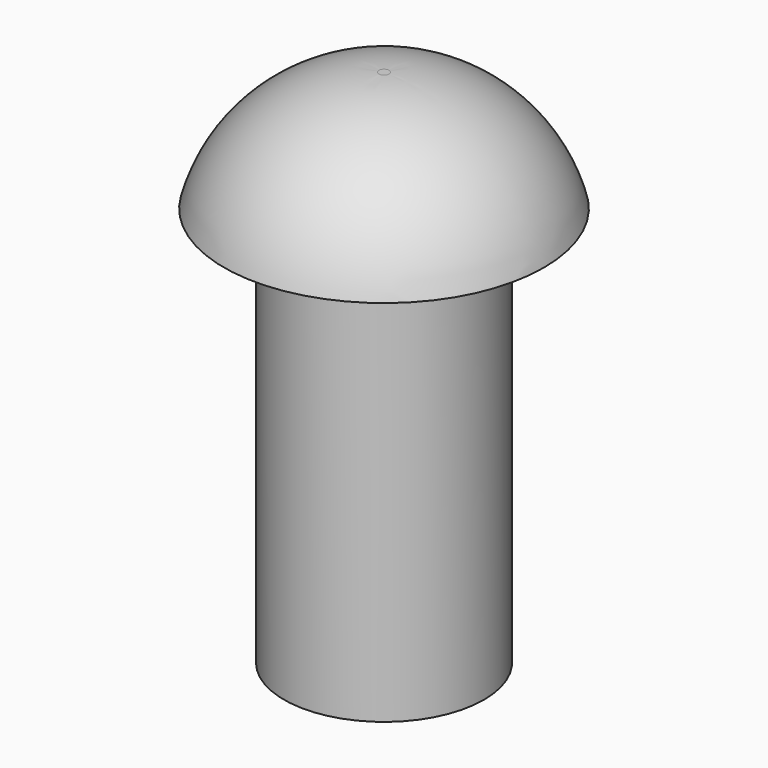
from build123d import *

# Parameters (mm, degrees)
F0_R     = 3.175
F1_DEPTH = 12.7
F2_R     = 5.08
F3_DEPTH = 3.81


# Not quite as in the source:
# - a fillet or chamfer that OpenCascade refuses, or shapes differently, is made with other operations: its cross-section is extruded or revolved along the edge and cut away or added


with BuildPart() as f1:
    # F0 (on Top) → F1 (new body)
    with BuildSketch(Plane.XY):
        with Locations((-67.7428916097, -29.48333323)):
            Circle(F0_R)
    extrude(amount=F1_DEPTH)

    # F2 (on face) → F3 (join)
    with BuildSketch(Plane.XY.offset(12.7)):
        with Locations((-67.7428916097, -29.48333323)):
            Circle(F2_R)
    extrude(amount=F3_DEPTH)

    # F4: fillet of radius 5.08 on 1 edges, made by hand

    # F4_s1 → F4_t2 (revolve, cut)
    with BuildSketch(Plane.XZ.offset(29.48333323)):
        with BuildLine():
            ThreePointArc((-62.6628916097, 12.7), (-64.470728486, 15.4460926284), (-67.5815804594, 16.51))
            Line((-67.5815804594, 16.51), (-62.6628916097, 16.51))
            Line((-62.6628916097, 16.51), (-62.6628916097, 12.7))
        make_face()
    revolve(axis=Axis((-67.7428916097, -29.48333323, 16.51), (0, 0, 1)), mode=Mode.SUBTRACT)


solid = f1.part
